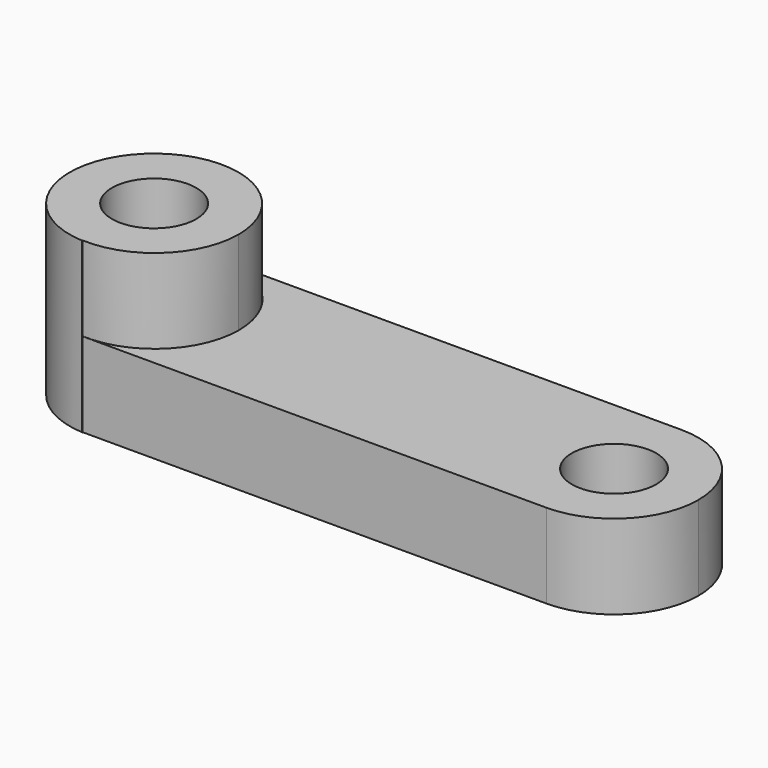
from build123d import *

# Parameters (mm, degrees)
F1_DEPTH = 12.7
F3_DEPTH = 25.4
F4_R     = 6.35
F5_DEPTH = 25.4
F6_R     = 6.35
F7_DEPTH = 12.7


with BuildPart() as f1:
    # F0 (on Top) → F1 (new body)
    with BuildSketch(Plane.XY):
        with BuildLine():
            ThreePointArc((-98.5095974419, 17.1447865009), (-89.9721430512, 13.1994974474), (-86.4897244217, 4.4630111011))
            ThreePointArc((-86.4897244217, 4.4630111011), (-90.4532380754, -4.7545702694), (-99.8698514014, -8.2187642987))
            Line((-99.8698514014, -8.2187642987), (-99.8698514014, -8.2552134991))
            Line((-99.8698514014, -8.2552134991), (-30.0198514014, -8.2552134991))
            ThreePointArc((-30.0198514014, -8.2552134991), (-42.7198514014, 4.4447865009), (-30.0198514014, 17.1447865009))
            Line((-30.0198514014, 17.1447865009), (-98.5095974419, 17.1447865009))
        make_face()
        with BuildLine():
            ThreePointArc((-17.3198514014, 4.4447865009), (-21.0395952804, 13.425042622), (-30.0198514014, 17.1447865009))
            Line((-30.0198514014, 17.1447865009), (-30.0198514014, -8.2552134991))
            ThreePointArc((-30.0198514014, -8.2552134991), (-21.0395952804, -4.5354696201), (-17.3198514014, 4.4447865009))
        make_face()
        with BuildLine():
            Line((-30.0198514014, -8.2552134991), (-30.0198514014, 17.1447865009))
            ThreePointArc((-30.0198514014, 17.1447865009), (-42.7198514014, 4.4447865009), (-30.0198514014, -8.2552134991))
        make_face()
    extrude(amount=F1_DEPTH)

    # F2 (on face) → F3 (join)
    with BuildSketch(Plane(origin=(0, 0, 0), x_dir=(1, 0, 0), z_dir=(0, 0, -1))):
        with BuildLine():
            ThreePointArc((-99.8698514014, -17.0553149368), (-90.4694861278, -13.6064937824), (-86.4898032129, -4.418275319))
            ThreePointArc((-86.4898032129, -4.418275319), (-90.4694861278, 4.7699431443), (-99.8698514014, 8.2187642987))
            Line((-99.8698514014, 8.2187642987), (-99.8698514014, -17.0553149368))
        make_face()
        with BuildLine():
            Line((-99.8698514014, 8.2187642987), (-99.8698514014, 8.2552134991))
            Line((-99.8698514014, 8.2552134991), (-99.8698514014, 8.3082358629))
            ThreePointArc((-99.8698514014, 8.3082358629), (-111.8897244217, -4.373539537), (-99.8698514014, -17.0553149368))
            Line((-99.8698514014, -17.0553149368), (-99.8698514014, 8.2187642987))
        make_face()
    extrude(amount=-F3_DEPTH)

    # F4 (on face) → F5 (cut)
    with BuildSketch(Plane.XY.offset(25.4)):
        with Locations((-99.1897244217, 4.373539537)):
            Circle(F4_R)
    extrude(amount=-F5_DEPTH, mode=Mode.SUBTRACT)

    # F6 (on face) → F7 (cut)
    with BuildSketch(Plane.XY.offset(12.7)):
        with Locations((-30.0198514014, 4.4447865009)):
            Circle(F6_R)
    extrude(amount=-F7_DEPTH, mode=Mode.SUBTRACT)


solid = f1.part
